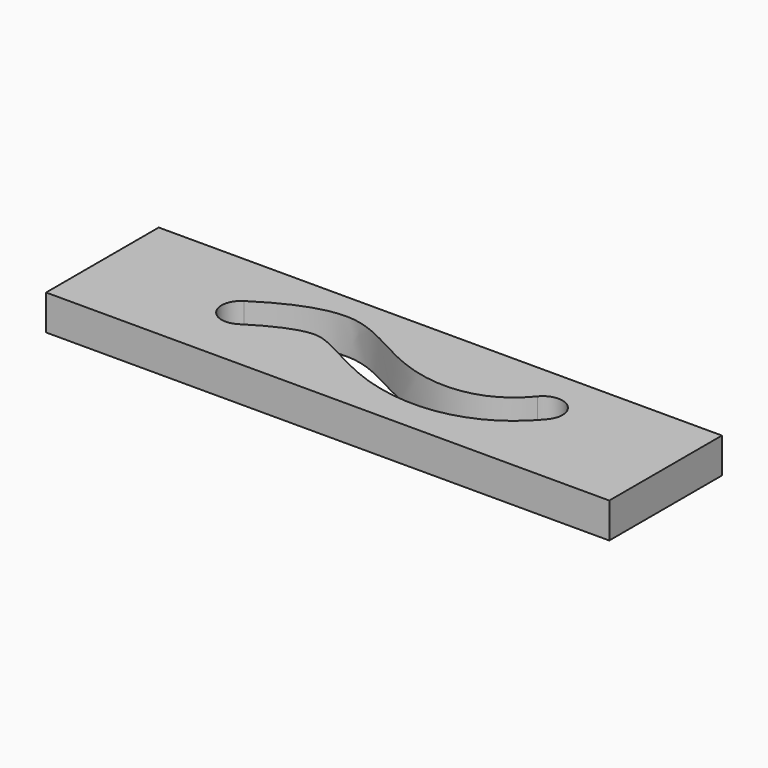
from build123d import *

# Parameters (mm, degrees)
F0_W     = 304.8
F0_H     = 76.2
F1_DEPTH = 19.05
F3_DEPTH = 19.051


# Not quite as in the source:
# - ends of sketch curves that miss each other by under 0.0002 mm in the source are joined
# - the dataset's text gives a spline's control points without its knots; the knots are read off the source's solid


with BuildPart() as f1:
    # F0 (on Top) → F1 (new body)
    with BuildSketch(Plane.XY):
        with Locations((152.4, -38.1)):
            Rectangle(F0_W, F0_H)
    extrude(amount=F1_DEPTH)

    # F2 (on face) → F3 (cut, through all)
    with BuildSketch(Plane.XY.offset(19.05)):
        with BuildLine():
            add(Edge.make_bspline(
                [(70.1576073312, -30.029141407), (83.8686786031, -21.2390518965), (117.9745576641, -3.9540702085), (159.6208902788, -40.3289545827), (205.6183690509, -40.2707766242), (221.5114043243, -20.7346916154)],
                knots=[0, 0, 0, 0, 0.3185426721, 0.6436291127, 1, 1, 1, 1], degree=3))
            ThreePointArc((70.1576073312, -30.029141407), (66.9343190895, -44.7676238402), (81.6727976161, -47.9909146072))
            add(Edge.make_bspline(
                [(81.6727976161, -47.9909146072), (84.0877078652, -46.4427239337), (87.7972943111, -44.1834375492), (92.7456157009, -41.5055188175), (96.4048002662, -39.7144739174), (99.953145037, -38.1869631858), (103.3238841372, -36.9617080625), (106.4437149489, -36.0649864483), (108.7706970233, -35.5977280038), (110.4345440663, -35.3818537852), (111.5775186819, -35.2932242999), (112.4393003762, -35.2746121128), (113.074386477, -35.2886281533), (113.4488140122, -35.3084633316), (113.7357681205, -35.3304787019), (114.0125672237, -35.3561984658), (114.3713475215, -35.3982021395), (114.823296753, -35.4655269195), (115.4584809497, -35.5797510491), (116.3184991054, -35.7719720031), (117.4672011442, -36.0925230731), (118.7373027036, -36.5115464684), (120.5934313466, -37.208525225), (123.2139088205, -38.3457103996), (126.8117272473, -40.1162505426), (130.8408991234, -42.2339963632), (135.2966060437, -44.6167638753), (140.1915298055, -47.1658672318), (144.6589639847, -49.3352302573), (148.4828140179, -51.0342568699), (151.47981133, -52.2727642861), (154.087858913, -53.2599589136), (156.242098264, -54.0129489576), (158.4198806242, -54.7318488314), (161.1914455398, -55.5668254183), (165.7252800795, -56.7556420347), (171.5733771699, -57.9455171062), (178.8563213148, -58.8226774722), (186.3740977432, -59.0583860083), (194.0825636932, -58.5480493219), (201.9140833068, -57.1765022895), (209.7666820369, -54.827878984), (217.4979195028, -51.4036396846), (224.9316159757, -46.8452266864), (231.8819965363, -41.1499646241), (236.0860264461, -36.6284650948), (238.062287508, -34.19919948)],
                knots=[0, 0, 0, 0, 0.0625, 0.09375, 0.125, 0.15625, 0.1875, 0.21875, 0.25, 0.265625, 0.28125, 0.296875, 0.3046875, 0.3125, 0.31640625, 0.3203125, 0.328125, 0.3359375, 0.34375, 0.359375, 0.375, 0.390625, 0.40625, 0.4375, 0.46875, 0.5, 0.53125, 0.5625, 0.59375, 0.609375, 0.625, 0.640625, 0.6484375, 0.65625, 0.671875, 0.6875, 0.71875, 0.75, 0.78125, 0.8125, 0.84375, 0.875, 0.90625, 0.9375, 0.96875, 1, 1, 1, 1], degree=3))
            ThreePointArc((238.062287508, -34.19919948), (236.5190998484, -19.1915039558), (221.5114043243, -20.7346916154))
        make_face()
    extrude(amount=-F3_DEPTH, mode=Mode.SUBTRACT)


solid = f1.part
